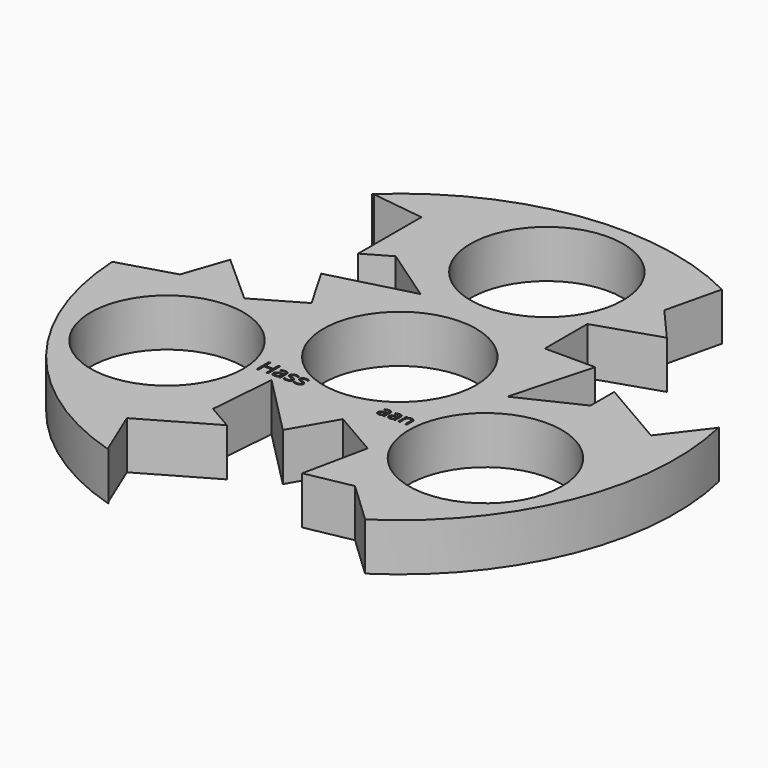
from build123d import *

# Parameters (mm, degrees)
F0_R         = 40.5133701228
F0_R_2       = 11.2
F1_DEPTH     = 7
F2_TEXT_SIZE = 3.0873436845
F3_DEPTH     = 0.51
F4_TEXT_SIZE = 2.8406800185
F5_DEPTH     = 0.64
F8_DEPTH     = 25


# Not quite as in the source:
# - Text() gives the source's letters only with a copy of the font that has no kerning and outlines rounded to 1/6400 em; it was checked with that copy


with BuildPart() as f1:
    # F0 (on Top) → F1 (new body)
    with BuildSketch(Plane.XY):
        Circle(F0_R)
        with Locations((-23.352673207, -13.4826721624)):
            Circle(F0_R_2, mode=Mode.SUBTRACT)
        with Locations((23.352673207, -13.4826721624)):
            Circle(F0_R_2, mode=Mode.SUBTRACT)
        Circle(F0_R_2, mode=Mode.SUBTRACT)
        with Locations((0, 26.9653443247)):
            Circle(F0_R_2, mode=Mode.SUBTRACT)
    extrude(amount=F1_DEPTH)

    # F2 (on face) → F3 (cut)
    with BuildSketch(Plane.XY.offset(7)):
        with Locations((-11.2112455724, -12.6004500012)):
            Text('Hass', F2_TEXT_SIZE, font='Open Sans', text_align=(TextAlign.LEFT, TextAlign.BOTTOM))
    extrude(amount=-F3_DEPTH, mode=Mode.SUBTRACT)

    # F4 (on face) → F5 (cut)
    with BuildSketch(Plane.XY.offset(7)):
        with Locations((6.4620403573, -12.6233948395)):
            Text('aan', F4_TEXT_SIZE, font='Open Sans', text_align=(TextAlign.LEFT, TextAlign.BOTTOM))
    extrude(amount=-F5_DEPTH, mode=Mode.SUBTRACT)

    # F7 (on face) → F8 (cut)
    with BuildSketch(Plane.XY.offset(7)):
        Polygon((44.1402904689, 32.3246233165), (18.4092260897, 36.2832471728), (16.4299122989, 27.9701352119), (20.9163539112, 22.8239223361), (11.6795636714, 19.7889767587), (11.6795636714, 12.0036816224), (19.0689973533, 12.0036816224), (15.7701410353, 0), (24.6110707521, 4.2183841579), (24.6110707521, 8.5728727281), (34.6395894885, 2.7668885887), (39.3899381161, 8.9687341824), align=None)
        Polygon((-27.4621206998, 29.6283199708), (-50.0640901943, 22.0643012183), (-40.6268268283, -2.1987661287), (-32.4378037903, 0.2436538268), (-30.2242735126, 6.7021326736), (-22.9775384236, 0.2203104651), (-16.2352750597, 4.1129580333), (-19.9299919006, 10.5123953214), (-7.8850705177, 13.6573427578), (-15.9587632197, 19.2046204068), (-19.729860942, 17.0273761216), (-19.7159905515, 28.6153201794), align=None)
        Polygon((-11.9278174163, -38.5970541532), (5.9237997254, -54.3889245348), (22.2176007386, -34.0844810441), (16.0078914914, -28.2137890388), (9.3079196015, -29.5260550097), (11.2979747523, -20.0092872239), (4.5557113883, -16.1166396557), (0.8609945473, -22.5160769439), (-7.8850705177, -13.6573427578), (-8.6523075324, -23.4230045646), (-4.8812098101, -25.6002488497), (-14.923598937, -31.382208768), align=None)
    extrude(amount=-F8_DEPTH, mode=Mode.SUBTRACT)


solid = f1.part
